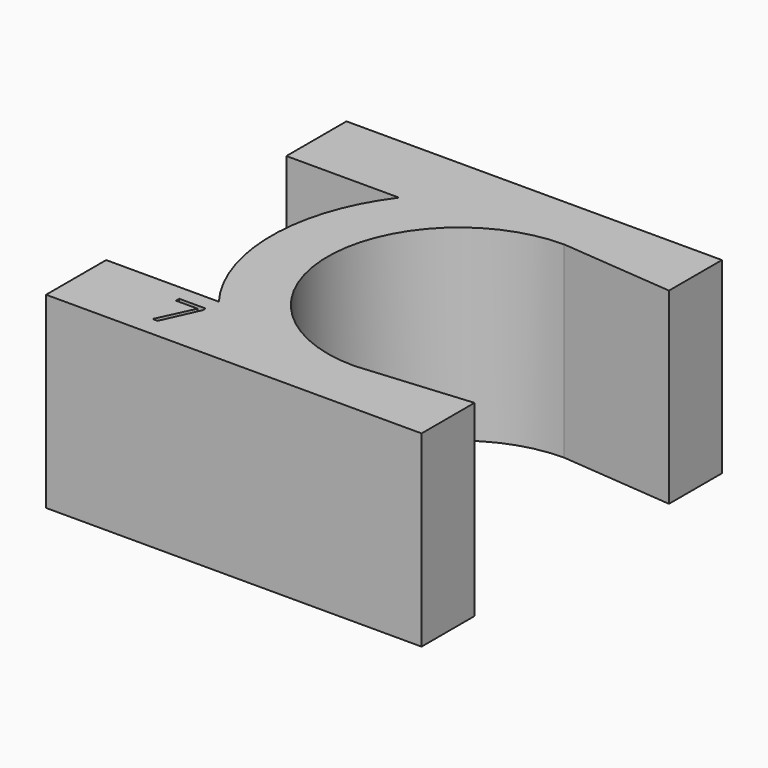
from build123d import *

# Parameters (mm, degrees)
F1_DEPTH     = 5
F2_TEXT_SIZE = 1.4821853256
F3_DEPTH     = 2


# Not quite as in the source:
# - Text() gives the source's letters only with a copy of the font that has no kerning and outlines rounded to 1/6400 em; it was checked with that copy


with BuildPart() as f1:
    # F0 (on Top) → F1 (new body)
    with BuildSketch(Plane.XY):
        with BuildLine():
            ThreePointArc((0, -3.5), (-3.5, 0), (0, 3.5))
            Line((0, 3.5), (3, 3.2375340094))
            Line((3, 3.2375340094), (3, 5))
            Line((3, 5), (0, 5))
            Line((0, 5), (-7, 5))
            Line((-7, 5), (-7, 3))
            Line((-7, 3), (-4, 3))
            ThreePointArc((-4, 3), (-5, 0), (-4, -3))
            Line((-4, -3), (-7, -3))
            Line((-7, -3), (-7, -5))
            Line((-7, -5), (0, -5))
            Line((0, -5), (3, -5))
            Line((3, -5), (3, -3.2375340094))
            Line((3, -3.2375340094), (0, -3.5))
        make_face()
    extrude(amount=F1_DEPTH)

    # F2 (on face) → F3 (cut)
    with BuildSketch(Plane.XY.offset(5)):
        with Locations((-4.792493768, -4.4698263519)):
            Text('7', F2_TEXT_SIZE, font='Open Sans', text_align=(TextAlign.LEFT, TextAlign.BOTTOM))
    extrude(amount=-F3_DEPTH, mode=Mode.SUBTRACT)


solid = f1.part
